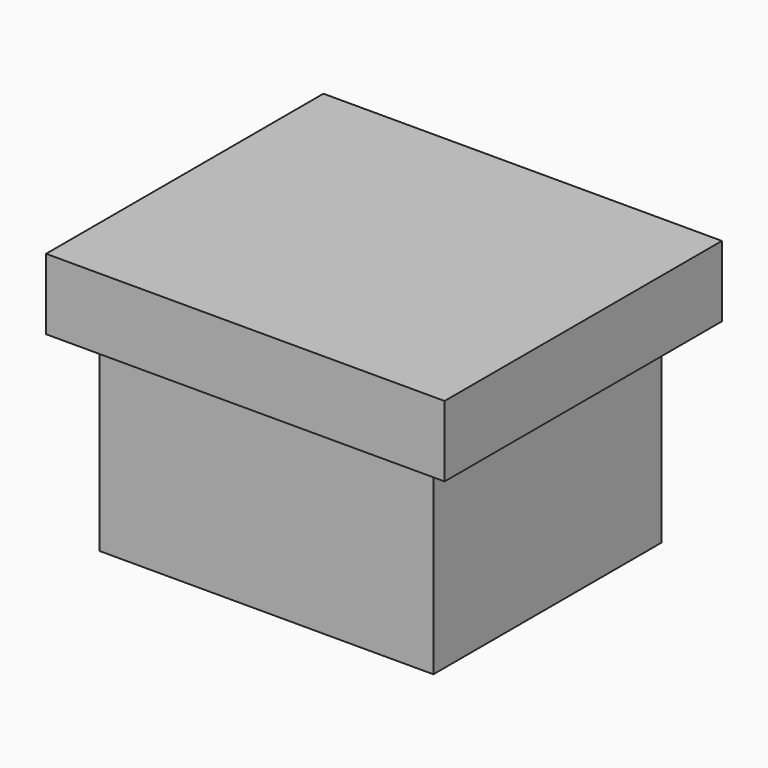
from build123d import *

# Parameters (mm, degrees)
F0_W     = 142.8329795599
F0_H     = 124.2600418627
F1_DEPTH = 25.4
F2_W     = 119.6952909231
F2_H     = 102.2856533527
F3_DEPTH = 67.056


# Not quite as in the source:
# - the program builds the solid bodies; features that only make, move or delete a surface that nothing else refers to are left out


with BuildPart() as f1:
    # F0 (on Top) → F1 (new body)
    with BuildSketch(Plane.XY):
        with Locations((-16.9922932982, 8.1018041819)):
            Rectangle(F0_W, F0_H)
    extrude(amount=F1_DEPTH)

    # F2 (on face) → F3 (join)
    with BuildSketch(Plane(origin=(0, 0, 0), x_dir=(1, 0, 0), z_dir=(0, 0, -1))):
        with Locations((-15.306442976, -4.4551417232)):
            Rectangle(F2_W, F2_H)
    extrude(amount=F3_DEPTH)


solid = f1.part
